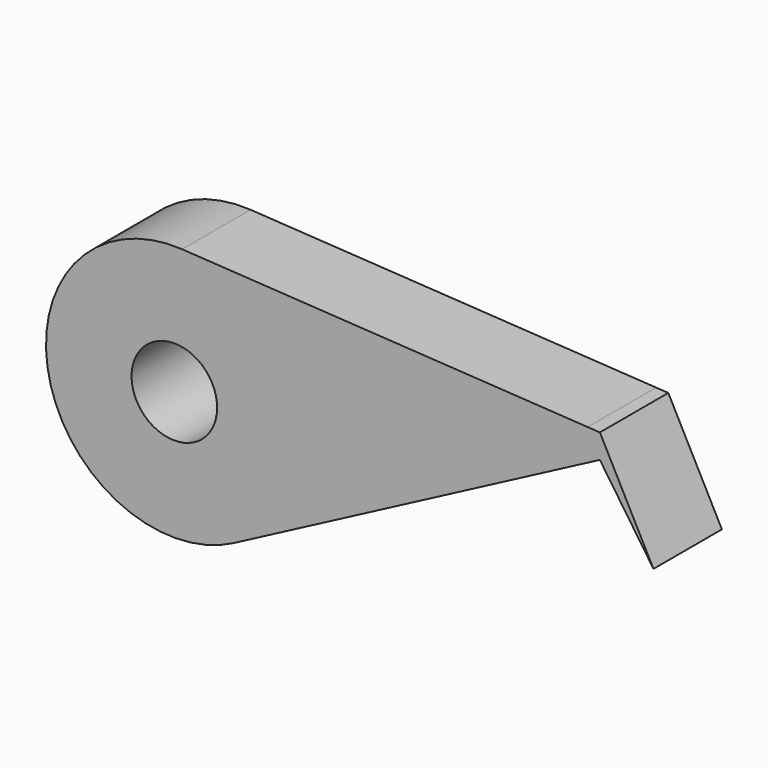
from build123d import *

# Parameters (mm, degrees)
F0_R     = 3.175
F1_DEPTH = 6.35


# Not quite as in the source:
# - the program builds the solid bodies; features that only make, move or delete a surface that nothing else refers to are left out


with BuildPart() as f1:
    # F0 (on Front) → F1 (new body)
    with BuildSketch(Plane.XZ):
        with BuildLine():
            ThreePointArc((4.4289185951, -8.4326926351), (8.1520265768, -4.9264680747), (9.525, 0))
            ThreePointArc((9.525, 0), (6.936415596, 6.5277686601), (0.5776480463, 9.5074679981))
            ThreePointArc((0.5776480463, 9.5074679981), (-9.3128281564, -1.9992140281), (4.4289185951, -8.4326926351))
        make_face()
        Circle(F0_R, mode=Mode.SUBTRACT)
        with BuildLine():
            ThreePointArc((0.5776480463, 9.5074679981), (6.936415596, 6.5277686601), (9.525, 0))
            ThreePointArc((9.525, 0), (8.1520265768, -4.9264680747), (4.4289185951, -8.4326926351))
            Line((4.4289185951, -8.4326926351), (20.4848255962, 0))
            Line((20.4848255962, 0), (31.5823644939, 5.8285174748))
            Line((31.5823644939, 5.8285174748), (35.56, 0))
            Line((35.56, 0), (31.5823644939, 7.623705267))
            Line((31.5823644939, 7.623705267), (30.6727180917, 7.6789729226))
            Line((30.6727180917, 7.6789729226), (0.5776480463, 9.5074679981))
        make_face()
    extrude(amount=F1_DEPTH)


solid = f1.part
